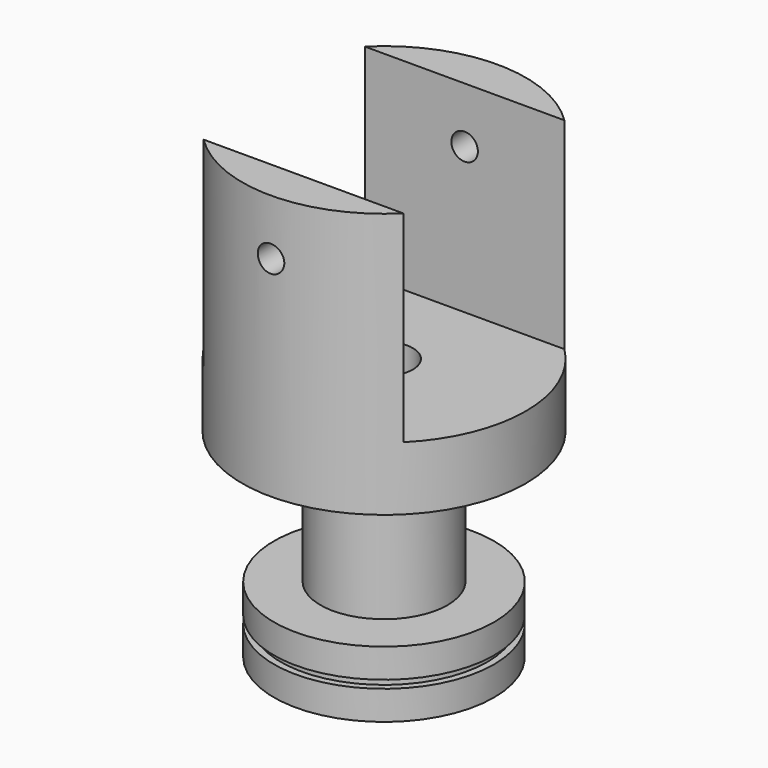
from build123d import *

# Parameters (mm, degrees)
F0_R      = 53.5
F0_R_2    = 10.9127793542
F1_DEPTH  = 100
F2_R      = 10.9127793542
F3_DEPTH  = 76
F5_R      = 23.9808815671
F5_R_2    = 10.9127793542
F6_DEPTH  = 50
F7_R      = 41.5
F7_R_2    = 23.9808815671
F7_R_3    = 10.9127793542
F8_DEPTH  = 11
F9_R      = 39
F9_R_2    = 10.9127793542
F10_DEPTH = 3
F11_R     = 41.5
F11_R_2   = 39
F11_R_3   = 10.9127793542
F12_DEPTH = 11
F13_R     = 5
F14_DEPTH = 125


# Not quite as in the source:
# - a feature names something its author has since deleted; it is built from what else it names


with BuildPart() as f1:
    # F0 (on Top) → F1 (new body)
    with BuildSketch(Plane.XY):
        Circle(F0_R)
        Circle(F0_R_2, mode=Mode.SUBTRACT)
    extrude(amount=F1_DEPTH)


with BuildPart() as f3:
    # F2 (on face) → F3 (new body)
    with BuildSketch(Plane.XY.offset(100)):
        with BuildLine():
            ThreePointArc((53.5, 0), (49.381382201, 20.5846810011), (37.6596601153, 38))
            Line((37.6596601153, 38), (-37.6596601153, 38))
            ThreePointArc((-37.6596601153, 38), (-53.5, 0), (-37.6596601153, -38))
            Line((-37.6596601153, -38), (37.6596601153, -38))
            ThreePointArc((37.6596601153, -38), (49.381382201, -20.5846810011), (53.5, 0))
        make_face()
        Circle(F2_R, mode=Mode.SUBTRACT)
    extrude(amount=-F3_DEPTH)


with BuildPart() as f1_1:
    add(f1.part)

    # F4: cut F3
    add(f3.part, mode=Mode.SUBTRACT)

    # F5 (on face) → F6 (join)
    with BuildSketch(Plane(origin=(0, 0, 0), x_dir=(1, 0, 0), z_dir=(0, 0, -1))):
        Circle(F5_R)
        Circle(F5_R_2, mode=Mode.SUBTRACT)
    extrude(amount=F6_DEPTH)

    # F7 (on face) → F8 (join)
    with BuildSketch(Plane(origin=(0, 0, -50), x_dir=(1, 0, 0), z_dir=(0, 0, -1))):
        Circle(F7_R)
        Circle(F7_R_2, mode=Mode.SUBTRACT)
        Circle(F7_R_2)
        Circle(F7_R_3, mode=Mode.SUBTRACT)
    extrude(amount=F8_DEPTH)

    # F9 (on face) → F10 (join)
    with BuildSketch(Plane(origin=(0, 0, -61), x_dir=(1, 0, 0), z_dir=(0, 0, -1))):
        Circle(F9_R)
        Circle(F9_R_2, mode=Mode.SUBTRACT)
    extrude(amount=F10_DEPTH)

    # F11 (on face) → F12 (join)
    with BuildSketch(Plane(origin=(0, 0, -64), x_dir=(1, 0, 0), z_dir=(0, 0, -1))):
        Circle(F11_R)
        Circle(F11_R_2, mode=Mode.SUBTRACT)
        Circle(F11_R_2)
        Circle(F11_R_3, mode=Mode.SUBTRACT)
    extrude(amount=F12_DEPTH)


with BuildPart() as f14:
    # F13 (on Front) → F14 (new body)
    with BuildSketch(Plane.XZ):
        with Locations((-63.11737746, -22.980183363)):
            Circle(F13_R)
    extrude(amount=F14_DEPTH)


with BuildPart() as f14_1:
    # F15: moved
    add(f14.part.moved(Location((63.12, 62.74391, 102))))


with BuildPart() as f1_2:
    add(f1_1.part)

    # F16: cut F14
    add(f14_1.part, mode=Mode.SUBTRACT)


solid = f1_2.part
